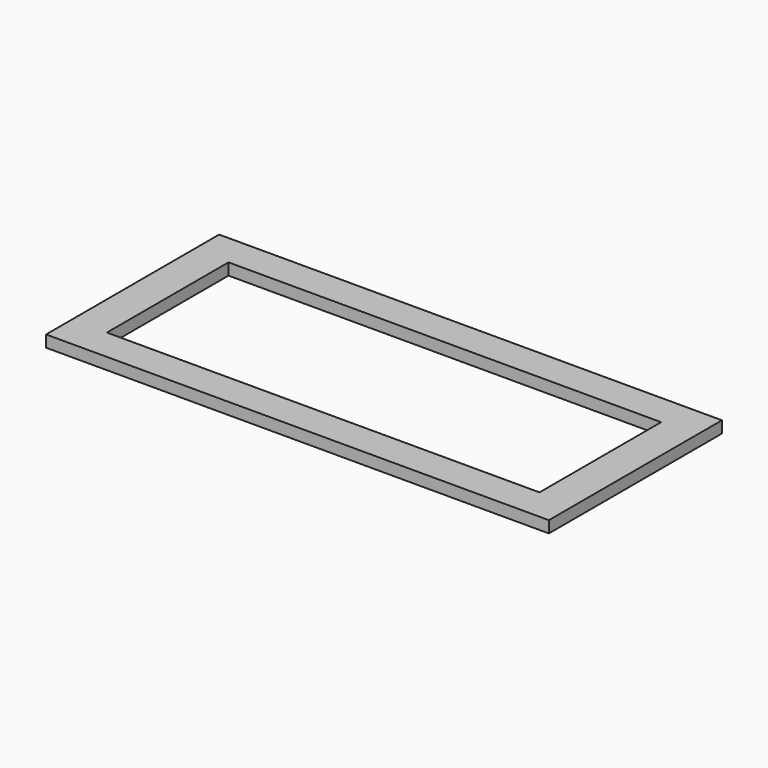
from build123d import *

# Parameters (mm, degrees)
F0_W     = 218.44
F0_H     = 93.98
F0_W_2   = 187.96
F0_H_2   = 66.04
F1_DEPTH = 5.08


with BuildPart() as f1:
    # F0 (on Top) → F1 (new body)
    with BuildSketch(Plane.XY):
        Rectangle(F0_W, F0_H)
        Rectangle(F0_W_2, F0_H_2, mode=Mode.SUBTRACT)
    extrude(amount=F1_DEPTH)


solid = f1.part
